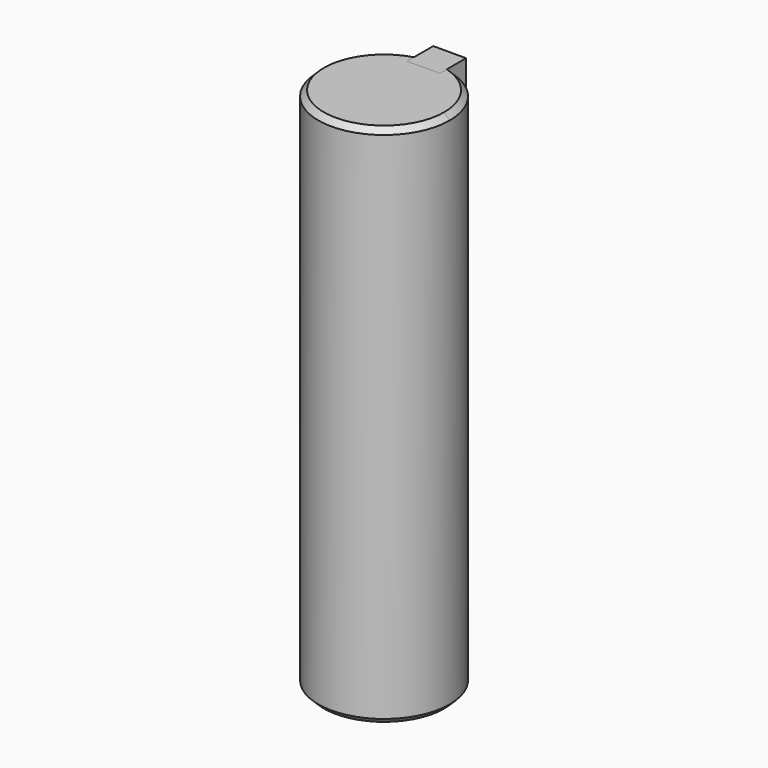
from build123d import *

# Parameters (mm, degrees)
F0_R     = 9.525
F1_DEPTH = 76.2
F3_DEPTH = 25.4
F4_R     = 2.38115
F5_W     = 4.7625
F5_H     = 23.01875
F6_DEPTH = 4.7625
F7_SIZE  = 0.79375


# Not quite as in the source:
# - a fillet or chamfer is up to 0.001 mm smaller than in the source, because OpenCascade refuses the exact size


with BuildPart() as f1:
    # F0 (on Top) → F1 (new body)
    with BuildSketch(Plane.XY):
        Circle(F0_R)
    extrude(amount=F1_DEPTH)

    # F2 (on face) → F3 (cut)
    with BuildSketch(Plane.XY.offset(76.2)):
        with BuildLine():
            ThreePointArc((2.38125, 9.2225415932), (0, 9.525), (-2.38125, 9.2225415932))
            Line((-2.38125, 9.2225415932), (-2.38125, 7.14375))
            Line((-2.38125, 7.14375), (2.38125, 7.14375))
            Line((2.38125, 7.14375), (2.38125, 9.2225415932))
        make_face()
    extrude(amount=-F3_DEPTH, mode=Mode.SUBTRACT)

    # F4 (radius 2.38125 in the source; OpenCascade refuses exactly that, so slightly less here)
    f4_edges = [f1.edges().sort_by_distance(p)[0] for p in [
        (2.38125, 8.183146, 50.8),
        (-2.38125, 8.183146, 50.8),
    ]]
    fillet(f4_edges, radius=F4_R)

    # F7
    f7_edges = [f1.edges().sort_by_distance(p)[0] for p in [
        (-5.832847, -7.530174, 76.2),
        (-9.525, 0, 0),
    ]]
    chamfer(f7_edges, length=F7_SIZE)


with BuildPart() as f6:
    # F5 (on face) → F6 (new body)
    with BuildSketch(Plane(origin=(0, 7.14375, 0), x_dir=(-1, 0, 0), z_dir=(0, 1, 0))):
        with Locations((0, 64.690625)):
            Rectangle(F5_W, F5_H)
    extrude(amount=F6_DEPTH)


solid = Compound([f1.part, f6.part])
